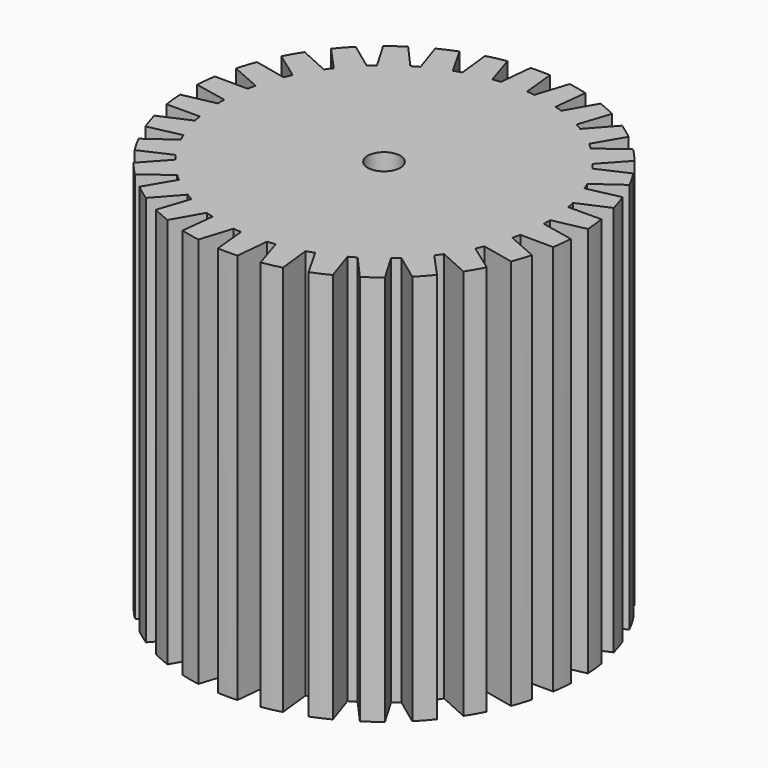
from build123d import *

# Parameters (mm, degrees)
F0_R            = 7.62
F1_DEPTH        = 7.62
F2_R            = 0.635
F3_DEPTH        = 15.24
F5_DEPTH        = 15.24
F5_COPIES_COUNT = 30


# Not quite as in the source:
# - a pattern or mirror of a feature is missing from the dataset's text; its kind, count and spacing are read off the source's solid


with BuildPart() as f1:
    # F0 (on Top) → F1 (new body, symmetric)
    with BuildSketch(Plane.XY):
        Circle(F0_R)
    extrude(amount=F1_DEPTH, both=True)

    # F2 (on face) → F3 (cut, through all)
    with BuildSketch(Plane.XY.offset(7.62)):
        Circle(F2_R)
    extrude(amount=-F3_DEPTH, mode=Mode.SUBTRACT)

    # F4 (on face) → F5 (cut, through all)
    with BuildSketch(Plane.XY.offset(7.62)):
        with BuildLine():
            ThreePointArc((1.20963125, 7.5233763856), (0.7965068901, 7.5782568427), (0.381, 7.6104690394))
            Line((0.381, 7.6104690394), (0.508, 6.3296473835))
            ThreePointArc((0.508, 6.3296473835), (0.6637557417, 6.3152140356), (0.8191087086, 6.2969485406))
            Line((0.8191087086, 6.2969485406), (1.20963125, 7.5233763856))
        make_face()
    f5 = extrude(amount=-F5_DEPTH, mode=Mode.SUBTRACT)

    # F5_copies: F5 ×30 about axis
    f5_copies_axis = Axis((0, 0, 0), (0, 0, 1))
    for i in range(1, F5_COPIES_COUNT):
        add(f5.rotate(f5_copies_axis, i * 360 / F5_COPIES_COUNT), mode=Mode.SUBTRACT)


solid = f1.part
